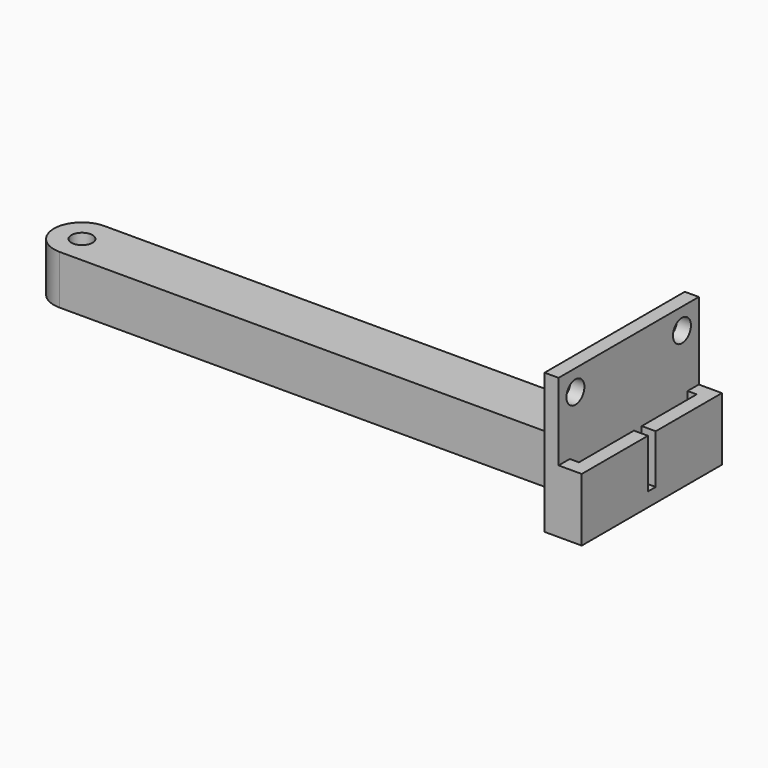
from build123d import *

# Parameters (mm, degrees)
F0_W     = 80
F0_H     = 8
F0_R     = 1.5
F1_DEPTH = 7
F2_R     = 3.99999
F3_W     = 25
F3_H     = 20
F4_DEPTH = 2
F6_DEPTH = 1.3
F8_DEPTH = 2
F9_D     = 3.2
F9_DEPTH = 6
F9_TIP   = 0.9613769904


# Not quite as in the source:
# - a fillet or chamfer is up to 0.001 mm smaller than in the source, because OpenCascade refuses the exact size


with BuildPart() as f1:
    # F0 (on Top) → F1 (new body)
    with BuildSketch(Plane.XY):
        with Locations((-23.5758614609, 11.990132276)):
            Rectangle(F0_W, F0_H)
        with Locations((-59.5758614609, 11.990132276)):
            Circle(F0_R, mode=Mode.SUBTRACT)
    extrude(amount=F1_DEPTH)

    # F2 (radius 4 in the source; OpenCascade refuses exactly that, so slightly less here)
    f2_edges = [f1.edges().sort_by_distance(p)[0] for p in [
        (-63.575861, 15.990132, 3.5),
        (-63.575861, 7.990132, 3.5),
    ]]
    fillet(f2_edges, radius=F2_R)

    # F3 (on face) → F4 (join)
    with BuildSketch(Plane.YZ.offset(16.4241385391)):
        with Locations((11.990132276, 10)):
            Rectangle(F3_W, F3_H)
    extrude(amount=F4_DEPTH)

    # F5 (on face) → F6 (join)
    with BuildSketch(Plane.YZ.offset(18.4241385391)):
        Polygon((1.490132276, 9), (-0.509867724, 9), (-0.509867724, 0), (24.490132276, 0), (24.490132276, 9), (22.490132276, 9), (22.490132276, 2), (1.490132276, 2), align=None)
    extrude(amount=F6_DEPTH)

    # F7 (on face) → F8 (join)
    with BuildSketch(Plane.YZ.offset(19.7241385391)):
        Polygon((11.290132276, 9), (-0.509867724, 9), (-0.509867724, 0), (24.490132276, 0), (24.490132276, 9), (12.690132276, 9), (12.690132276, 2), (11.290132276, 2), align=None)
    extrude(amount=F8_DEPTH)

    # F9
    with Locations(Plane(origin=(16.4241385391, 0, 0), x_dir=(0, 1, 0), z_dir=(-1, 0, 0))):
        with Locations((2.490132276, -17), (21.490132276, -17)):
            Hole(F9_D / 2, depth=F9_DEPTH)
            with Locations((0, 0, -(F9_DEPTH + F9_TIP / 2))):  # 118° drill point
                Cone(0, F9_D / 2, F9_TIP, mode=Mode.SUBTRACT)


solid = f1.part
